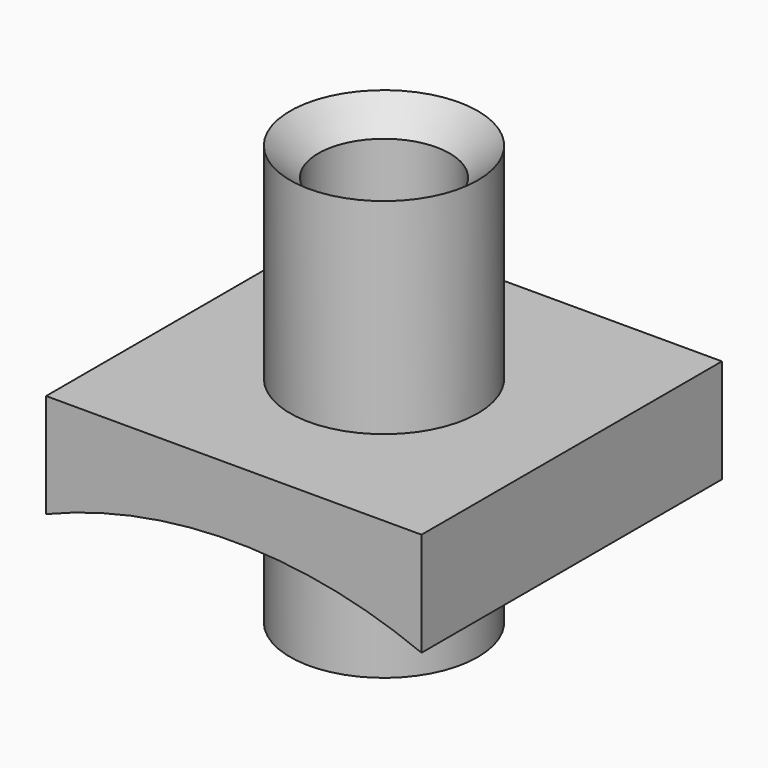
from build123d import *

# Parameters (mm, degrees)
F0_W     = 17.78
F0_H     = 17.78
F1_DEPTH = 7.62
F3_W     = 5.08
F3_H     = 22.724437993
F5_R     = 4.445
F5_R_2   = 3.1115
F6_DEPTH = 10.16
F7_DEPTH = 25.4
F8_DEPTH = 10.16


# Not quite as in the source:
# - a fillet or chamfer that OpenCascade refuses, or shapes differently, is made with other operations: its cross-section is extruded or revolved along the edge and cut away or added


with BuildPart() as f1:
    # F0 (on Top) → F1 (new body)
    with BuildSketch(Plane.XY):
        with Locations((8.89, 8.89)):
            Rectangle(F0_W, F0_H)
    extrude(amount=F1_DEPTH)

    # F3 (on offset) → F4 (revolve, cut)
    with BuildSketch(Plane(origin=(0, 0, -19.05), x_dir=(1, 0, 0), z_dir=(0, 0, -1))):
        with Locations((-12.065, -8.8908823673)):
            Rectangle(F3_W, F3_H)
    revolve(axis=Axis((8.89, 12.1113763889, -19.05), (0, 1, 0)), mode=Mode.SUBTRACT)

    # F5 (on face) → F6 (join)
    with BuildSketch(Plane.XY.offset(7.62)):
        with Locations((8.89, 8.89)):
            Circle(F5_R)
        with Locations((8.89, 8.89)):
            Circle(F5_R_2, mode=Mode.SUBTRACT)
    extrude(amount=F6_DEPTH)

    # F7 (cut): a face of the model
    f7_faces = [f1.faces().sort_by_distance(p)[0] for p in [
        (8.89, 8.89, 7.62),
    ]]
    extrude(f7_faces, amount=-F7_DEPTH, mode=Mode.SUBTRACT)

    # F5 (on face) → F8 (join)
    with BuildSketch(Plane.XY.offset(7.62)):
        with Locations((8.89, 8.89)):
            Circle(F5_R)
        with Locations((8.89, 8.89)):
            Circle(F5_R_2, mode=Mode.SUBTRACT)
    extrude(amount=-F8_DEPTH)

    # F9: chamfer of 1.778 on 1 edges, made by hand

    # F9_s1 → F9_t2 (revolve, cut)
    with BuildSketch(Plane.XZ.offset(-8.89)):
        Polygon((13.7795, 17.78), (12.0015, 16.002), (12.0015, 17.78), align=None)
    revolve(axis=Axis((8.89, 8.89, 17.78), (0, 0, 1)), mode=Mode.SUBTRACT)


solid = f1.part
